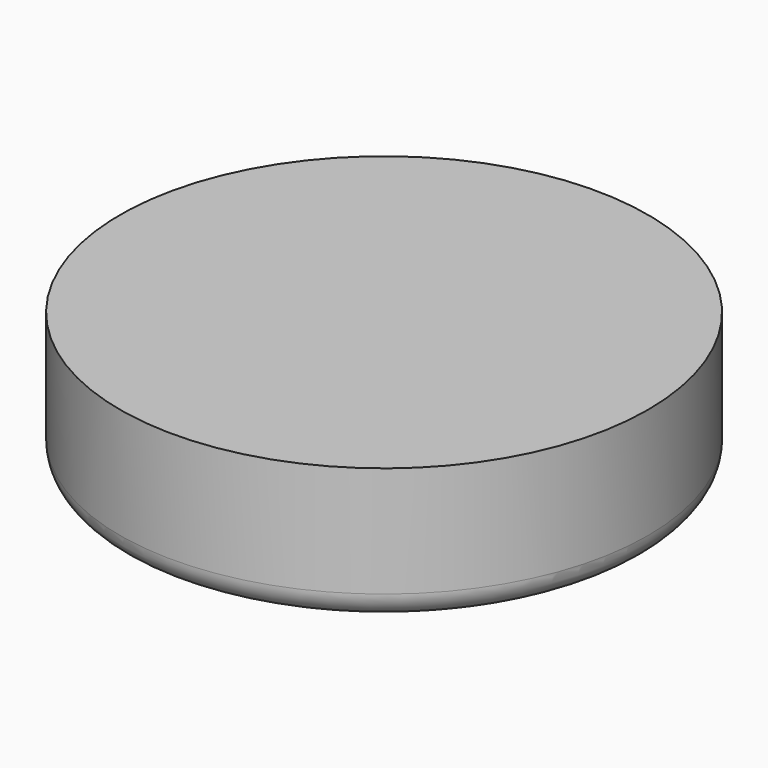
from build123d import *

# Parameters (mm, degrees)
F0_R     = 15.5
F1_DEPTH = 8
F2_T     = -5
F3_R     = 1.5
F4_R     = 1.2


with BuildPart() as f1:
    # F0 (on Top) → F1 (new body)
    with BuildSketch(Plane.XY):
        with Locations((-16.122315079, 8.5424212739)):
            Circle(F0_R)
    extrude(amount=F1_DEPTH)

    # F2
    f2_openings = [f1.faces().sort_by_distance(p)[0] for p in [
        (-16.122315, 8.542421, 0),
    ]]
    offset(amount=F2_T, openings=f2_openings)

    # F3
    f3_edges = [f1.edges().sort_by_distance(p)[0] for p in [
        (-31.622315, 8.542421, 0),
    ]]
    fillet(f3_edges, radius=F3_R)

    # F4
    f4_edges = [f1.edges().sort_by_distance(p)[0] for p in [
        (-26.622315, 8.542421, 0),
        (-1.061655, 8.542421, 0.43934),
        (-31.622315, 8.542421, 1.5),
        (-30.122315, 8.542421, 0),
    ]]
    fillet(f4_edges, radius=F4_R)


solid = f1.part
